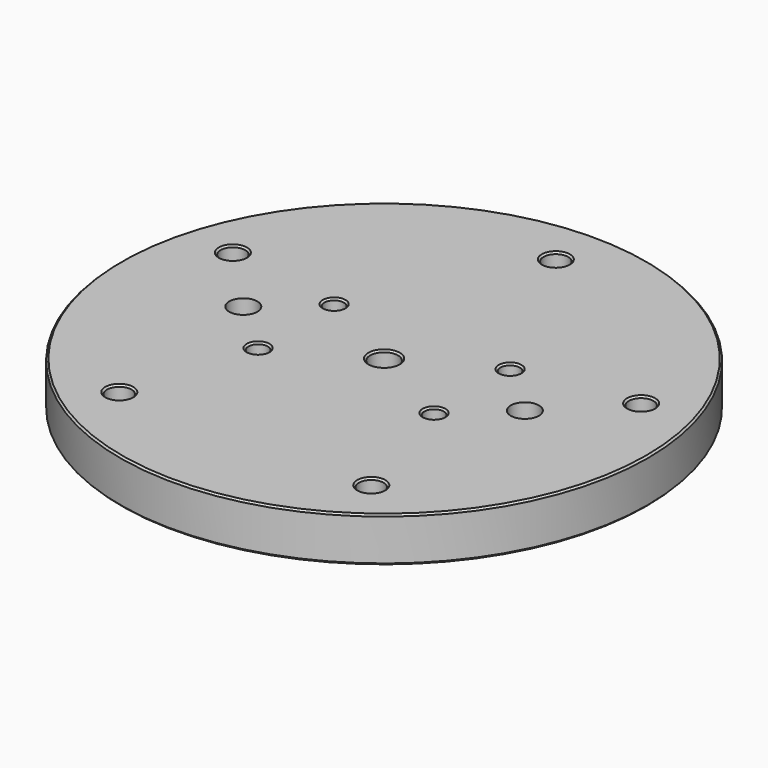
from build123d import *

# Parameters (mm, degrees)
F0_R           = 75
F1_DEPTH       = 12.7
F2_D           = 5.5
F2_CSINK_D     = 11.2
F2_CSINK_ANGLE = 90
F4_D           = 7
F5_D           = 7.9375
F8_D           = 8


# Not quite as in the source:
# - a fillet or chamfer that OpenCascade refuses, or shapes differently, is made with other operations: its cross-section is extruded or revolved along the edge and cut away or added
# - a length typed as a fraction of an inch, garbled in the dataset ("3 / 203.2 mm" for 3/8 in), is restored


with BuildPart() as f1:
    # F0 (on Top) → F1 (new body)
    with BuildSketch(Plane.XY):
        Circle(F0_R)
    extrude(amount=F1_DEPTH)

    # F2 (through all)
    with Locations(Plane(origin=(0, 0, 0), x_dir=(1, 0, 0), z_dir=(0, 0, -1))):
        with Locations((-25, 13.5), (25, 13.5), (-25, -13.5), (25, -13.5)):
            CounterSinkHole(F2_D / 2, F2_CSINK_D / 2, counter_sink_angle=F2_CSINK_ANGLE)

    # F4 (through all)
    with Locations(Plane.XY.offset(12.7)):
        with Locations((0, 61), (58, 18.8), (-58, 18.8), (-35.8, -49.3), (35.8, -49.3)):
            Hole(F4_D / 2)

    # F5 (through all)
    with Locations(Plane(origin=(0, 0, 0), x_dir=(1, 0, 0), z_dir=(0, 0, -1))):
        with Locations((0, 0)):
            Hole(F5_D / 2)

    # F6: chamfer of 0.5 on 22 edges, made by hand

    # F6_s1 → F6_t2 (revolve, cut)
    with BuildSketch(Plane.XZ):
        Polygon((75, 0.5), (74.5, 0), (75, 0), align=None)
    revolve(axis=Axis((0, 0, 0), (0, 0, 1)), mode=Mode.SUBTRACT)

    # F6_s3 → F6_t4 (revolve, cut)
    with BuildSketch(Plane.XZ.offset(49.3)):
        Polygon((-31.8, 0), (-32.3, 0.5), (-32.3, 0), align=None)
    revolve(axis=Axis((-35.8, -49.3, 0), (0, 0, 1)), mode=Mode.SUBTRACT)

    # F6_s5 → F6_t6 (revolve, cut)
    with BuildSketch(Plane.XZ.offset(13.5)):
        Polygon((-19.1938414904, 0), (-19.5474568916, 0.1465086309), (-19.4009996492, 0), align=None)
    revolve(axis=Axis((-25, -13.5, 0), (0, 0, -1)), mode=Mode.SUBTRACT)

    # F6_s7 → F6_t8 (revolve, cut)
    with BuildSketch(Plane.XZ.offset(49.3)):
        Polygon((39.8, 0), (39.3, 0.5), (39.3, 0), align=None)
    revolve(axis=Axis((35.8, -49.3, 0), (0, 0, 1)), mode=Mode.SUBTRACT)

    # F6_s9 → F6_t10 (revolve, cut)
    with BuildSketch(Plane.XZ.offset(13.5)):
        Polygon((30.8061585096, 0), (30.4525431084, 0.1465086309), (30.5990003508, 0), align=None)
    revolve(axis=Axis((25, -13.5, 0), (0, 0, -1)), mode=Mode.SUBTRACT)

    # F6_s11 → F6_t12 (revolve, cut)
    with BuildSketch(Plane.XZ):
        Polygon((4.46875, 0), (3.96875, 0.5), (3.96875, 0), align=None)
    revolve(axis=Axis((0, 0, 0), (0, 0, -1)), mode=Mode.SUBTRACT)

    # F6_s13 → F6_t14 (revolve, cut)
    with BuildSketch(Plane.XZ.offset(-18.8)):
        Polygon((-54, 0), (-54.5, 0.5), (-54.5, 0), align=None)
    revolve(axis=Axis((-58, 18.8, 0), (0, 0, 1)), mode=Mode.SUBTRACT)

    # F6_s15 → F6_t16 (revolve, cut)
    with BuildSketch(Plane.XZ.offset(-13.5)):
        Polygon((-19.1938414904, 0), (-19.5474568916, 0.1465086309), (-19.4009996492, 0), align=None)
    revolve(axis=Axis((-25, 13.5, 0), (0, 0, -1)), mode=Mode.SUBTRACT)

    # F6_s17 → F6_t18 (revolve, cut)
    with BuildSketch(Plane.XZ.offset(-13.5)):
        Polygon((30.8061585096, 0), (30.4525431084, 0.1465086309), (30.5990003508, 0), align=None)
    revolve(axis=Axis((25, 13.5, 0), (0, 0, -1)), mode=Mode.SUBTRACT)

    # F6_s19 → F6_t20 (revolve, cut)
    with BuildSketch(Plane.XZ.offset(-18.8)):
        Polygon((62, 0), (61.5, 0.5), (61.5, 0), align=None)
    revolve(axis=Axis((58, 18.8, 0), (0, 0, 1)), mode=Mode.SUBTRACT)

    # F6_s21 → F6_t22 (revolve, cut)
    with BuildSketch(Plane.XZ.offset(-61)):
        Polygon((4, 0), (3.5, 0.5), (3.5, 0), align=None)
    revolve(axis=Axis((0, 61, 0), (0, 0, 1)), mode=Mode.SUBTRACT)

    # F6_s23 → F6_t24 (revolve, cut)
    with BuildSketch(Plane.XZ):
        Polygon((75, 12.2), (74.5, 12.7), (75, 12.7), align=None)
    revolve(axis=Axis((0, 0, 12.7), (0, 0, 1)), mode=Mode.SUBTRACT)

    # F6_s25 → F6_t26 (revolve, cut)
    with BuildSketch(Plane.XZ.offset(49.3)):
        Polygon((-31.8, 12.7), (-32.3, 12.2), (-32.3, 12.7), align=None)
    revolve(axis=Axis((-35.8, -49.3, 12.7), (0, 0, 1)), mode=Mode.SUBTRACT)

    # F6_s27 → F6_t28 (revolve, cut)
    with BuildSketch(Plane.XZ.offset(13.5)):
        Polygon((-21.75, 12.7), (-22.25, 12.2), (-22.25, 12.7), align=None)
    revolve(axis=Axis((-25, -13.5, 12.7), (0, 0, -1)), mode=Mode.SUBTRACT)

    # F6_s29 → F6_t30 (revolve, cut)
    with BuildSketch(Plane.XZ.offset(49.3)):
        Polygon((39.8, 12.7), (39.3, 12.2), (39.3, 12.7), align=None)
    revolve(axis=Axis((35.8, -49.3, 12.7), (0, 0, 1)), mode=Mode.SUBTRACT)

    # F6_s31 → F6_t32 (revolve, cut)
    with BuildSketch(Plane.XZ.offset(13.5)):
        Polygon((28.25, 12.7), (27.75, 12.2), (27.75, 12.7), align=None)
    revolve(axis=Axis((25, -13.5, 12.7), (0, 0, -1)), mode=Mode.SUBTRACT)

    # F6_s33 → F6_t34 (revolve, cut)
    with BuildSketch(Plane.XZ):
        Polygon((4.46875, 12.7), (3.96875, 12.2), (3.96875, 12.7), align=None)
    revolve(axis=Axis((0, 0, 12.7), (0, 0, -1)), mode=Mode.SUBTRACT)

    # F6_s35 → F6_t36 (revolve, cut)
    with BuildSketch(Plane.XZ.offset(-18.8)):
        Polygon((-54, 12.7), (-54.5, 12.2), (-54.5, 12.7), align=None)
    revolve(axis=Axis((-58, 18.8, 12.7), (0, 0, 1)), mode=Mode.SUBTRACT)

    # F6_s37 → F6_t38 (revolve, cut)
    with BuildSketch(Plane.XZ.offset(-13.5)):
        Polygon((-21.75, 12.7), (-22.25, 12.2), (-22.25, 12.7), align=None)
    revolve(axis=Axis((-25, 13.5, 12.7), (0, 0, -1)), mode=Mode.SUBTRACT)

    # F6_s39 → F6_t40 (revolve, cut)
    with BuildSketch(Plane.XZ.offset(-13.5)):
        Polygon((28.25, 12.7), (27.75, 12.2), (27.75, 12.7), align=None)
    revolve(axis=Axis((25, 13.5, 12.7), (0, 0, -1)), mode=Mode.SUBTRACT)

    # F6_s41 → F6_t42 (revolve, cut)
    with BuildSketch(Plane.XZ.offset(-18.8)):
        Polygon((62, 12.7), (61.5, 12.2), (61.5, 12.7), align=None)
    revolve(axis=Axis((58, 18.8, 12.7), (0, 0, 1)), mode=Mode.SUBTRACT)

    # F6_s43 → F6_t44 (revolve, cut)
    with BuildSketch(Plane.XZ.offset(-61)):
        Polygon((4, 12.7), (3.5, 12.2), (3.5, 12.7), align=None)
    revolve(axis=Axis((0, 61, 12.7), (0, 0, 1)), mode=Mode.SUBTRACT)

    # F8 (through all)
    with Locations(Plane.XY.offset(12.7)):
        with Locations((-40, 0), (40, 0)):
            Hole(F8_D / 2)


solid = f1.part
